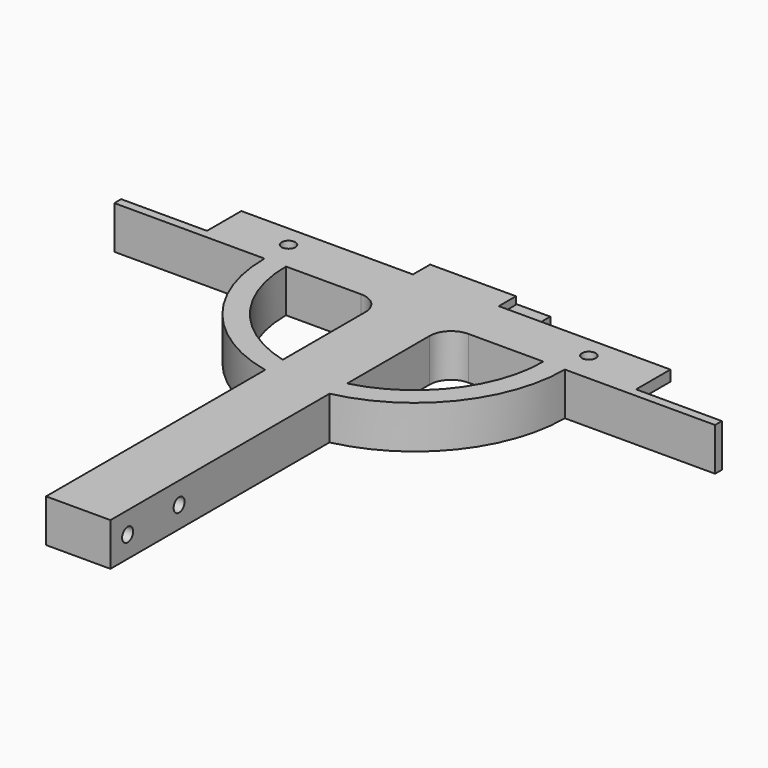
from build123d import *

# Parameters (mm, degrees)
F0_W      = 15
F0_H      = 100
F1_DEPTH  = 5
F2_W      = 100
F2_H      = 10
F3_DEPTH  = 10
F4_W      = 10
F4_H      = 5
F5_DEPTH  = 20
F6_W      = 10
F6_H      = 5
F7_DEPTH  = 20
F8_R      = 1.6
F9_DEPTH  = 10
F10_W     = 77.5
F10_H     = 10
F10_W_2   = 140
F11_DEPTH = 2
F12_R     = 5
F13_R     = 1.6
F14_DEPTH = 15
F15_W     = 20
F15_H     = 10
F16_DEPTH = 5
F17_W     = 20
F17_H     = 6.5
F18_DEPTH = 3
F19_DEPTH = 10
F21_DEPTH = 10


# Not quite as in the source:
# - a pattern or mirror of a feature is missing from the dataset's text; its kind, count and spacing are read off the source's solid


with BuildPart() as f1:
    # F0 (on Top) → F1 (new body, symmetric)
    with BuildSketch(Plane.XY):
        Rectangle(F0_W, F0_H)
    extrude(amount=F1_DEPTH, both=True)

    # F2 (on face) → F3 (join)
    with BuildSketch(Plane(origin=(0, 50, 0), x_dir=(-1, 0, 0), z_dir=(0, 1, 0))):
        Rectangle(F2_W, F2_H)
    extrude(amount=F3_DEPTH)

    # F4 (on face) → F5 (cut)
    with BuildSketch(Plane(origin=(-50, 0, 0), x_dir=(0, -1, 0), z_dir=(-1, 0, 0))):
        with Locations((-55, 0)):
            Rectangle(F4_W, F4_H)
    extrude(amount=-F5_DEPTH, mode=Mode.SUBTRACT)

    # F6 (on face) → F7 (cut)
    with BuildSketch(Plane.YZ.offset(50)):
        with Locations((55, 0)):
            Rectangle(F6_W, F6_H)
    extrude(amount=-F7_DEPTH, mode=Mode.SUBTRACT)

    # F8 (on face) → F9 (cut, through all)
    with BuildSketch(Plane.XY.offset(5)):
        with Locations((-35, 55)):
            Circle(F8_R)
        with Locations((35, 55)):
            Circle(F8_R)
    extrude(amount=-F9_DEPTH, mode=Mode.SUBTRACT)

    # F10 (on face) → F11 (join)
    with BuildSketch(Plane.XZ.offset(-50)):
        with Locations((31.25, 0)):
            Rectangle(F10_W, F10_H)
        Rectangle(F10_W_2, F10_H)
    extrude(amount=F11_DEPTH)

    # F12
    f12_edges = [f1.edges().sort_by_distance(p)[0] for p in [
        (-7.5, 48, 0),
        (7.5, 48, 0),
    ]]
    fillet(f12_edges, radius=F12_R)

    # F13 (on face) → F14 (cut, through all)
    with BuildSketch(Plane(origin=(-7.5, 0, 0), x_dir=(0, -1, 0), z_dir=(-1, 0, 0))):
        with Locations((30, 0)):
            Circle(F13_R)
        with Locations((45, 0)):
            Circle(F13_R)
    extrude(amount=-F14_DEPTH, mode=Mode.SUBTRACT)

    # F15 (on face) → F16 (join)
    with BuildSketch(Plane(origin=(0, 60, 0), x_dir=(-1, 0, 0), z_dir=(0, 1, 0))):
        Rectangle(F15_W, F15_H)
    extrude(amount=F16_DEPTH)

    # F17 (on face) → F18 (cut)
    with BuildSketch(Plane(origin=(0, 65, 0), x_dir=(-1, 0, 0), z_dir=(0, 1, 0))):
        Rectangle(F17_W, F17_H)
    extrude(amount=-F18_DEPTH, mode=Mode.SUBTRACT)

    # F19 (add): a face of the model
    f19_faces = [f1.faces().sort_by_distance(p)[0] for p in [
        (0, 65, -4.125),
    ]]
    extrude(f19_faces, amount=F19_DEPTH)

    # F20 (on face) → F21 (join, through all)
    with BuildSketch(Plane.XY.offset(5)):
        with BuildLine():
            Line((35, 48), (30, 48))
            ThreePointArc((30, 48), (23.7170824513, 29.6288269291), (7.5, 18.9526249034))
            Line((7.5, 18.9526249034), (7.5, 13.8130141721))
            ThreePointArc((7.5, 13.8130141721), (27.2717802866, 26.0625890315), (35, 48))
        make_face()
    f21 = extrude(amount=-F21_DEPTH)

    # F21_copies: F21 across plane
    add(f21.mirror(Plane(origin=(0, 0, 0), x_dir=(0, 0, -1), z_dir=(-1, 0, 0))))


solid = f1.part
